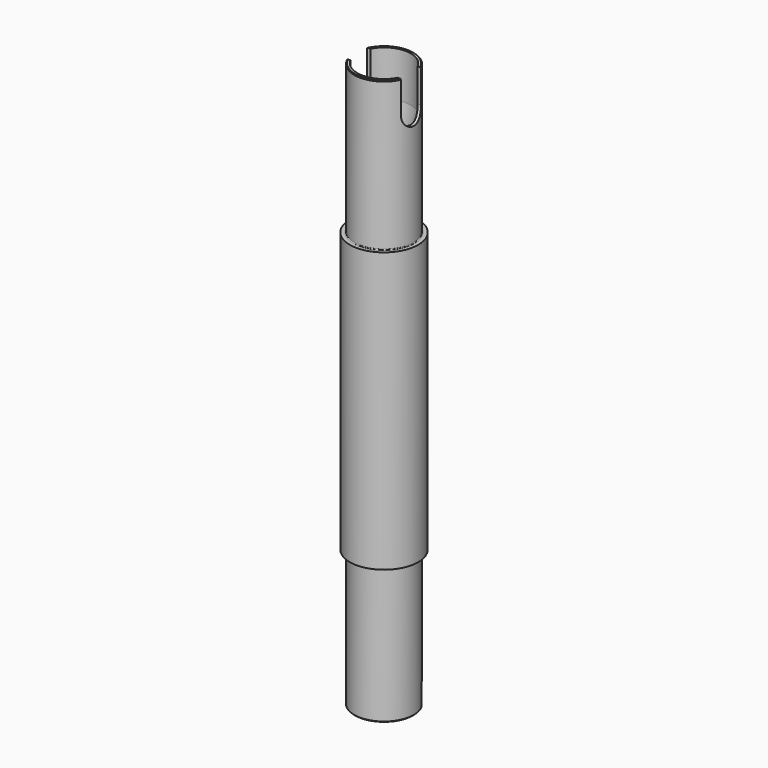
from build123d import *

# Parameters (mm, degrees)
F0_R      = 11.25
F0_R_2    = 9.8
F1_DEPTH  = 46
F0_R_3    = 5.3
F2_DEPTH  = 80
F3_SIZE2  = 20
F3_SIZE   = 3.5
F4_SIZE2  = 20
F4_SIZE   = 3.5
F6_DEPTH  = 11
F7_DEPTH  = 25
F8_DEPTH  = 15
F9_R      = 0.25
F10_SIZE  = 0.24999
F11_R     = 0.25
F13_DEPTH = 25


# Not quite as in the source:
# - a fillet or chamfer is up to 0.001 mm smaller than in the source, because OpenCascade refuses the exact size


with BuildPart() as f1:
    # F0 (on Top) → F1 (new body, symmetric)
    with BuildSketch(Plane.XY):
        Circle(F0_R)
        Circle(F0_R_2, mode=Mode.SUBTRACT)
    extrude(amount=F1_DEPTH, both=True)

    # F0 (on Top) → F2 (join, symmetric)
    with BuildSketch(Plane.XY):
        Circle(F0_R_2)
        Circle(F0_R_3, mode=Mode.SUBTRACT)
    extrude(amount=F2_DEPTH, both=True)

    # F3
    f3_edges = [f1.edges().sort_by_distance(p)[0] for p in [
        (-5.3, 0, 80),
    ]]
    f3_side = f1.faces().sort_by_distance((-9.522814, 0, 80))[0]
    chamfer(f3_edges, length=F3_SIZE, length2=F3_SIZE2, reference=f3_side)

    # F4
    f4_edges = [f1.edges().sort_by_distance(p)[0] for p in [
        (-5.3, 0, -80),
    ]]
    f4_side = f1.faces().sort_by_distance((-9.522814, 0, -80))[0]
    chamfer(f4_edges, length=F4_SIZE, length2=F4_SIZE2, reference=f4_side)

    # F6 (add): a face of the model
    f6_faces = [f1.faces().sort_by_distance(p)[0] for p in [
        (-9.0771858582, 0, -80),
    ]]
    extrude(f6_faces, amount=F6_DEPTH)

    # F5 (on Front) → F7 (cut)
    with BuildSketch(Plane.XZ):
        with BuildLine():
            Line((0, -84), (8, -84))
            ThreePointArc((8, -84), (0, -76), (-8, -84))
            Line((-8, -84), (0, -84))
        make_face()
        with BuildLine():
            ThreePointArc((-8, -84), (0, -92), (8, -84))
            Line((8, -84), (0, -84))
            Line((0, -84), (-8, -84))
        make_face()
        with BuildLine():
            Line((8, -104.4733112454), (8, -84))
            ThreePointArc((8, -84), (0, -92), (-8, -84))
            Line((-8, -84), (-8, -104.4733112454))
            Line((-8, -104.4733112454), (8, -104.4733112454))
        make_face()
    extrude(amount=-F7_DEPTH, mode=Mode.SUBTRACT)

    # F8 (add): a face of the model
    f8_faces = [f1.faces().sort_by_distance(p)[0] for p in [
        (-9.0771858582, 0, 80),
    ]]
    extrude(f8_faces, amount=F8_DEPTH)

    # F9
    f9_edges = [f1.edges().sort_by_distance(p)[0] for p in [
        (0, 9.8, -76),
    ]]
    fillet(f9_edges, radius=F9_R)

    # F10 (size 0.25 in the source; OpenCascade refuses exactly that, so slightly less here)
    f10_edges = [f1.edges().sort_by_distance(p)[0] for p in [
        (-2.556708, -9.460616, -91),
        (9.460616, 2.556708, -91),
        (-9.8, 0, 95),
    ]]
    chamfer(f10_edges, length=F10_SIZE)

    # F11
    f11_edges = [f1.edges().sort_by_distance(p)[0] for p in [
        (-9.8, 0, 46),
        (-9.8, 0, -46),
    ]]
    fillet(f11_edges, radius=F11_R)

    # F12 (on Right) → F13 (cut, symmetric)
    with BuildSketch(Plane.YZ):
        with BuildLine():
            ThreePointArc((-4.1, 84.1), (-2.8991378029, 81.2008621971), (0, 80))
            ThreePointArc((0, 80), (2.8991378029, 81.2008621971), (4.1, 84.1))
            ThreePointArc((4.1, 84.1), (0, 88.2), (-4.1, 84.1))
        make_face()
        with BuildLine():
            ThreePointArc((-4.1, 84.1), (0, 88.2), (4.1, 84.1))
            Line((4.1, 84.1), (4.1, 110))
            Line((4.1, 110), (-4.1, 110))
            Line((-4.1, 110), (-4.1, 84.1))
        make_face()
    extrude(amount=F13_DEPTH, both=True, mode=Mode.SUBTRACT)


solid = f1.part
